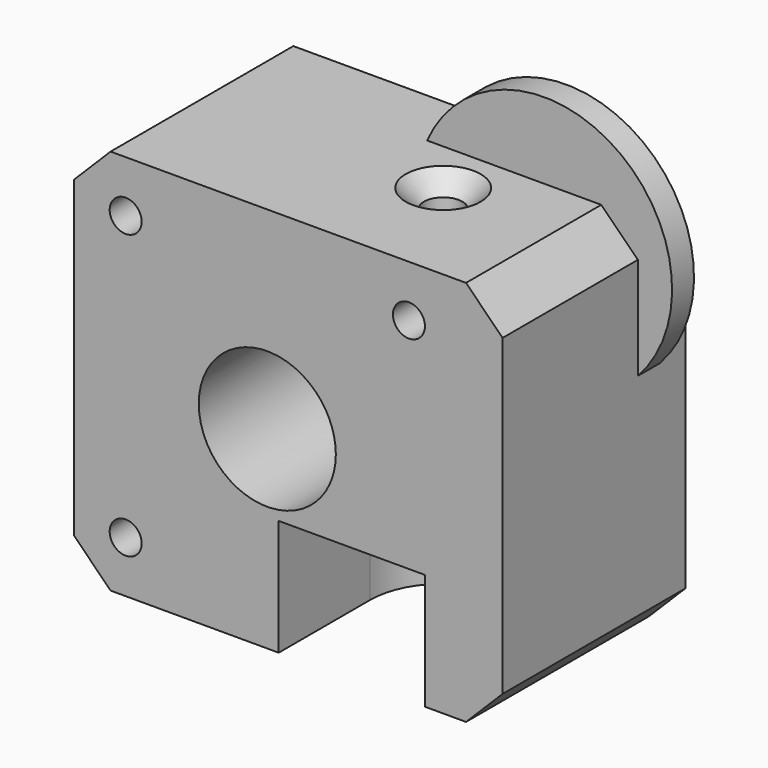
from build123d import *

# Parameters (mm, degrees)
F0_W      = 46.9
F0_H      = 42.3
F0_R      = 1.75
F1_DEPTH  = 25
F2_SIZE   = 4
F4_DEPTH  = 12.7
F5_R      = 2.1
F6_DEPTH  = 29.601
F7_SIZE   = 2
F9_DEPTH  = 25.0010001
F11_R     = 14
F12_DEPTH = 1.5


# Not quite as in the source:
# - a feature names something its author has since deleted; it is built from what else it names


with BuildPart() as f1:
    # F0 (on Front) → F1 (new body)
    with BuildSketch(Plane.XZ):
        Rectangle(F0_W, F0_H)
        with Locations((-17.8, -15.5)):
            Circle(F0_R, mode=Mode.SUBTRACT)
        with Locations((13.2, -15.5)):
            Circle(F0_R, mode=Mode.SUBTRACT)
        with Locations((-17.8, 15.5)):
            Circle(F0_R, mode=Mode.SUBTRACT)
        with Locations((13.2, 15.5)):
            Circle(F0_R, mode=Mode.SUBTRACT)
    extrude(amount=F1_DEPTH)

    # F2
    f2_edges = [f1.edges().sort_by_distance(p)[0] for p in [
        (-23.45, -12.5, 21.15),
        (23.45, -12.5, 21.15),
        (23.45, -12.5, -21.15),
        (-23.45, -12.5, -21.15),
    ]]
    chamfer(f2_edges, length=F2_SIZE)

    # F3 (on face) → F4 (cut)
    with BuildSketch(Plane(origin=(0, 0, -21.15), x_dir=(1, 0, 0), z_dir=(0, 0, -1))):
        with BuildLine():
            Line((6.95, 12.5), (14.95, 12.5))
            ThreePointArc((14.95, 12.5), (6.95, 20.5), (-1.05, 12.5))
            Line((-1.05, 12.5), (6.95, 12.5))
        make_face()
        with BuildLine():
            ThreePointArc((-1.05, 12.5), (6.95, 4.5), (14.95, 12.5))
            Line((14.95, 12.5), (6.95, 12.5))
            Line((6.95, 12.5), (-1.05, 12.5))
        make_face()
        with BuildLine():
            ThreePointArc((-1.05, 12.5), (6.95, 20.5), (14.95, 12.5))
            Line((14.95, 12.5), (14.95, 25))
            Line((14.95, 25), (-1.05, 25))
            Line((-1.05, 25), (-1.05, 12.5))
        make_face()
    extrude(amount=-F4_DEPTH, mode=Mode.SUBTRACT)

    # F5 (on face) → F6 (cut, through all)
    with BuildSketch(Plane(origin=(0, 0, -8.45), x_dir=(1, 0, 0), z_dir=(0, 0, -1))):
        with Locations((6.95, 12.5)):
            Circle(F5_R)
    extrude(amount=-F6_DEPTH, mode=Mode.SUBTRACT)

    # F7
    f7_edges = [f1.edges().sort_by_distance(p)[0] for p in [
        (4.85, -12.5, -8.45),
        (4.85, -12.5, 21.15),
    ]]
    chamfer(f7_edges, length=F7_SIZE)

    # F8 (on face) → F9 (cut, through all)
    with BuildSketch(Plane.XZ.offset(25)):
        with BuildLine():
            Line((-16.05, 15.5), (-17.8, 15.5))
            Line((-17.8, 15.5), (-16.5625631329, 14.2625631329))
            ThreePointArc((-16.5625631329, 14.2625631329), (-16.1832108181, 14.8303039934), (-16.05, 15.5))
        make_face()
        with BuildLine():
            Line((13.2, 15.5), (11.45, 15.5))
            ThreePointArc((11.45, 15.5), (11.5832108181, 14.8303039934), (11.9625631329, 14.2625631329))
            Line((11.9625631329, 14.2625631329), (13.2, 15.5))
        make_face()
        with BuildLine():
            ThreePointArc((-16.05, -15.5), (-16.1832108181, -14.8303039934), (-16.5625631329, -14.2625631329))
            Line((-16.5625631329, -14.2625631329), (-17.8, -15.5))
            Line((-17.8, -15.5), (-16.05, -15.5))
        make_face()
        with BuildLine():
            Line((3.0033008589, 5.3033008589), (-2.3, 0))
            Line((-2.3, 0), (3.0033008589, -5.3033008589))
            ThreePointArc((3.0033008589, -5.3033008589), (4.6290964938, -2.8701257427), (5.2, 0))
            ThreePointArc((5.2, 0), (4.6290964938, 2.8701257427), (3.0033008589, 5.3033008589))
        make_face()
        with BuildLine():
            ThreePointArc((3.0033008589, 5.3033008589), (-2.3, 7.5), (-7.6033008589, 5.3033008589))
            Line((-7.6033008589, 5.3033008589), (-2.3, 0))
            Line((-2.3, 0), (3.0033008589, 5.3033008589))
        make_face()
        with BuildLine():
            Line((-2.3, 0), (-7.6033008589, 5.3033008589))
            ThreePointArc((-7.6033008589, 5.3033008589), (-9.8, 0), (-7.6033008589, -5.3033008589))
            Line((-7.6033008589, -5.3033008589), (-2.3, 0))
        make_face()
        with BuildLine():
            Line((3.0033008589, -5.3033008589), (-2.3, 0))
            Line((-2.3, 0), (-7.6033008589, -5.3033008589))
            ThreePointArc((-7.6033008589, -5.3033008589), (-2.3, -7.5), (3.0033008589, -5.3033008589))
        make_face()
    extrude(amount=-F9_DEPTH, mode=Mode.SUBTRACT)

    # F11 (on offset) → F12 (join, symmetric)
    with BuildSketch(Plane.XZ.offset(5)):
        with Locations((13.2, 15.5)):
            Circle(F11_R)
    extrude(amount=F12_DEPTH, both=True)


solid = f1.part
